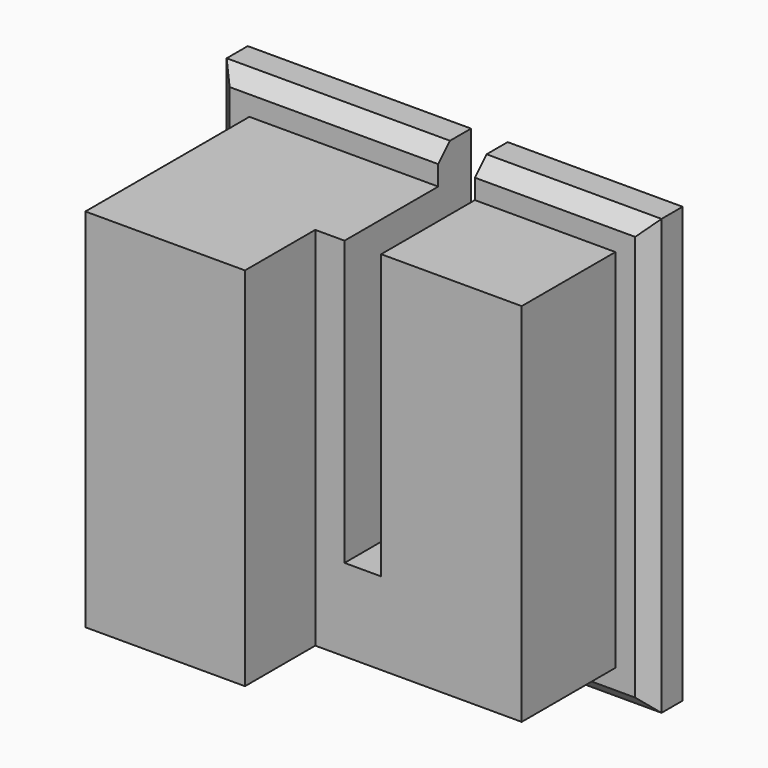
from build123d import *

# Parameters (mm, degrees)
F0_W      = 37.719
F0_H      = 37.719
F1_DEPTH  = 2.794
F2_W      = 31.75
F2_H      = 31.75
F3_DEPTH  = 10.16
F4_SIZE   = 1.27
F5_W      = 13.843
F5_H      = 31.75
F6_DEPTH  = 7.62
F7_W      = 3.175
F7_H      = 24.6046739221
F7_H_2    = 3.0808845013
F8_DEPTH  = 12.955
F9_W      = 3.1516091073
F9_H      = 27.5891739221
F10_DEPTH = 20.575
F11_DEPTH = 0.762


# Not quite as in the source:
# - a feature names something its author has since deleted; it is built from what else it names


with BuildPart() as f1:
    # F0 (on Front) → F1 (new body)
    with BuildSketch(Plane.XZ):
        Rectangle(F0_W, F0_H)
    extrude(amount=F1_DEPTH)

    # F2 (on face) → F3 (join)
    with BuildSketch(Plane.XZ.offset(2.794)):
        Rectangle(F2_W, F2_H)
    extrude(amount=F3_DEPTH)

    # F4
    f4_edges = [f1.edges().sort_by_distance(p)[0] for p in [
        (-18.8595, -2.794, 0),
        (0, -2.794, -18.8595),
        (18.8595, -2.794, 0),
        (0, -2.794, 18.8595),
    ]]
    chamfer(f4_edges, length=F4_SIZE)

    # F5 (on face) → F6 (join)
    with BuildSketch(Plane.XZ.offset(12.954)):
        with Locations((-8.9535, 0)):
            Rectangle(F5_W, F5_H)
    extrude(amount=F6_DEPTH)

    # F7 (on face) → F8 (cut, through all)
    with BuildSketch(Plane.XZ.offset(12.954)):
        with Locations((2.0955, 3.572663039)):
            Rectangle(F7_W, F7_H)
        with Locations((2.0955, 17.4154422507)):
            Rectangle(F7_W, F7_H_2)
    extrude(amount=-F8_DEPTH, mode=Mode.SUBTRACT)

    # F9 (on face) → F10 (cut, through all)
    with BuildSketch(Plane(origin=(0, 0, 0), x_dir=(-1, 0, 0), z_dir=(0, 1, 0))):
        with Locations((-2.0838045536, 5.064913039)):
            Rectangle(F9_W, F9_H)
    extrude(amount=-F10_DEPTH, mode=Mode.SUBTRACT)

    # F11 (add): a face of the model
    f11_faces = [f1.faces().sort_by_distance(p)[0] for p in [
        (-0.1374824949, 0, -0.3323010646),
    ]]
    extrude(f11_faces, amount=F11_DEPTH)


solid = f1.part
